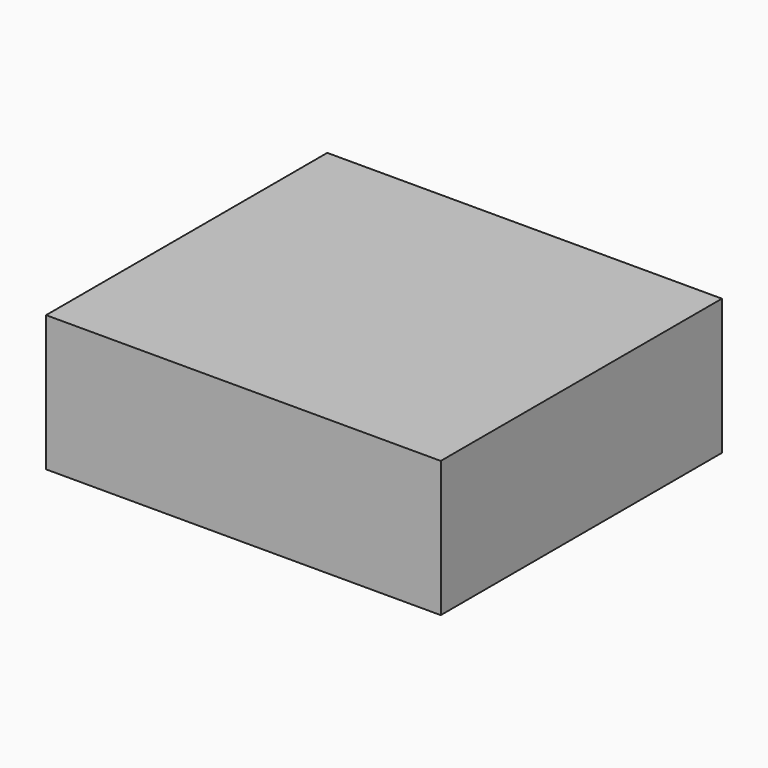
from build123d import *

# Parameters (mm, degrees)
F1_E0_TOP_W = 73.8316476345
F1_E0_TOP_H = 25.4
F2_DEPTH    = 65.7457243651


with BuildPart() as f2:
    # F1_E0_top (on explicit) → F2 (new body)
    with BuildSketch(Plane(origin=(-35.2146029472, -44.2385077477, -12.7), x_dir=(1, 0, 0), z_dir=(0, -1, 0))):
        with Locations((36.9158238173, 12.7)):
            Rectangle(F1_E0_TOP_W, F1_E0_TOP_H)
    extrude(amount=-F2_DEPTH)


solid = f2.part
